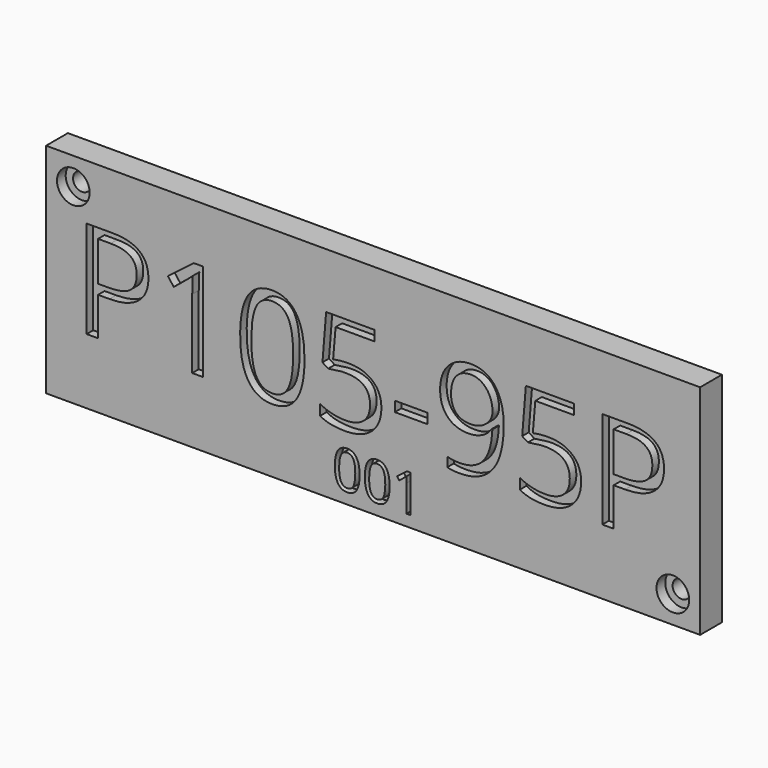
from build123d import *

# Parameters (mm, degrees)
F0_W           = 120
F0_H           = 40
F1_DEPTH       = 5
F3_D           = 3.3
F3_CBORE_D     = 6
F3_CBORE_DEPTH = 2
F5_D           = 3.3
F5_CBORE_D     = 6
F5_CBORE_DEPTH = 2
F6_TEXT_SIZE   = 25.0115465236
F7_DEPTH       = 1.5
F8_TEXT_SIZE   = 9.6317848901
F9_DEPTH       = 1.5


# Not quite as in the source:
# - Text() gives the source's letters only with a copy of the font that has no kerning and outlines rounded to 1/6400 em; it was checked with that copy


with BuildPart() as f1:
    # F0 (on Front) → F1 (new body)
    with BuildSketch(Plane.XZ):
        Rectangle(F0_W, F0_H)
    extrude(amount=F1_DEPTH)

    # F3 (through all)
    with Locations(Plane.XZ.offset(5)):
        with Locations((-55, 15)):
            CounterBoreHole(F3_D / 2, F3_CBORE_D / 2, F3_CBORE_DEPTH)

    # F5 (through all)
    with Locations(Plane.XZ.offset(5)):
        with Locations((55, -15)):
            CounterBoreHole(F5_D / 2, F5_CBORE_D / 2, F5_CBORE_DEPTH)

    # F6 (on face) → F7 (cut)
    with BuildSketch(Plane.XZ.offset(5)):
        with Locations((-55, -8.008313497)):
            Text('P105-95P', F6_TEXT_SIZE, font='Open Sans', text_align=(TextAlign.LEFT, TextAlign.BOTTOM))
    extrude(amount=-F7_DEPTH, mode=Mode.SUBTRACT)

    # F8 (on face) → F9 (cut)
    with BuildSketch(Plane.XZ.offset(5)):
        with Locations((-7.5, -17.9348851209)):
            Text('001', F8_TEXT_SIZE, font='Open Sans', text_align=(TextAlign.LEFT, TextAlign.BOTTOM))
    extrude(amount=-F9_DEPTH, mode=Mode.SUBTRACT)


solid = f1.part
